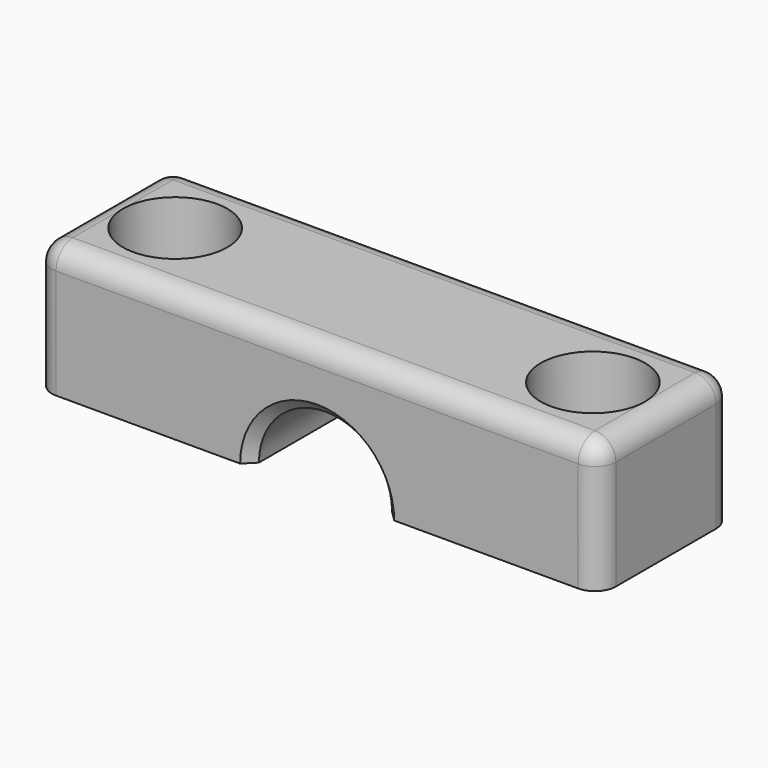
from build123d import *

# Parameters (mm, degrees)
F1_DEPTH = 16
F3_DEPTH = 12.501
F4_R     = 5
F4_R_2   = 2.75
F5_DEPTH = 6
F6_SIZE  = 1
F7_R     = 2
F8_R     = 1.99999


# Not quite as in the source:
# - a fillet or chamfer is up to 0.001 mm smaller than in the source, because OpenCascade refuses the exact size


with BuildPart() as f1:
    # F0 (on Front) → F1 (new body)
    with BuildSketch(Plane.XZ):
        with BuildLine():
            Line((27, 12.5), (-27, 12.5))
            Line((-27, 12.5), (-27, 0))
            Line((-27, 0), (-6.375, 0))
            ThreePointArc((-6.375, 0), (0, 6.375), (6.375, 0))
            Line((6.375, 0), (27, 0))
            Line((27, 0), (27, 12.5))
        make_face()
    extrude(amount=F1_DEPTH)

    # F2 (on face) → F3 (cut, through all)
    with BuildSketch(Plane.XY.offset(12.5)):
        with BuildLine():
            Line((-22.75, -8), (-17.25, -8))
            ThreePointArc((-17.25, -8), (-20, -5.25), (-22.75, -8))
        make_face()
        with BuildLine():
            ThreePointArc((-22.75, -8), (-20, -10.75), (-17.25, -8))
            Line((-17.25, -8), (-22.75, -8))
        make_face()
        with BuildLine():
            Line((17.25, -8), (22.75, -8))
            ThreePointArc((22.75, -8), (20, -5.25), (17.25, -8))
        make_face()
        with BuildLine():
            ThreePointArc((17.25, -8), (20, -10.75), (22.75, -8))
            Line((22.75, -8), (17.25, -8))
        make_face()
    extrude(amount=-F3_DEPTH, mode=Mode.SUBTRACT)

    # F4 (on face) → F5 (cut)
    with BuildSketch(Plane.XY.offset(12.5)):
        with Locations((-20, -8)):
            Circle(F4_R)
        with Locations((-20, -8)):
            Circle(F4_R_2, mode=Mode.SUBTRACT)
        with Locations((20, -8)):
            Circle(F4_R)
        with Locations((20, -8)):
            Circle(F4_R_2, mode=Mode.SUBTRACT)
    extrude(amount=-F5_DEPTH, mode=Mode.SUBTRACT)

    # F6
    f6_edges = [f1.edges().sort_by_distance(p)[0] for p in [
        (0, -16, 6.375),
        (0, 0, 6.375),
    ]]
    chamfer(f6_edges, length=F6_SIZE)

    # F7
    f7_edges = [f1.edges().sort_by_distance(p)[0] for p in [
        (27, 0, 6.25),
        (27, -16, 6.25),
        (-27, 0, 6.25),
        (-27, -16, 6.25),
    ]]
    fillet(f7_edges, radius=F7_R)

    # F8 (radius 2 in the source; OpenCascade refuses exactly that, so slightly less here)
    f8_edges = [f1.edges().sort_by_distance(p)[0] for p in [
        (0, 0, 12.5),
    ]]
    fillet(f8_edges, radius=F8_R)


solid = f1.part
